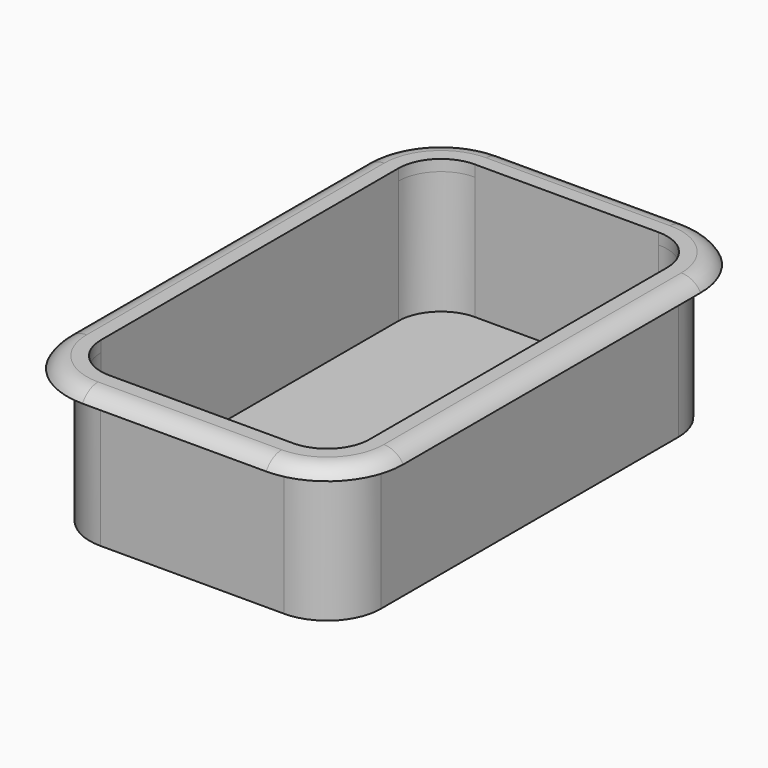
from build123d import *

# Parameters (mm, degrees)
F1_DEPTH     = 30
F2_T         = -2.5
F4_DEPTH     = 2.5
F5_T1_DEPTH  = 83
F5_T3_DEPTH  = 41
F5_T6_ANGLE  = 90
F5_T8_ANGLE  = 90
F5_T10_ANGLE = 90
F5_T12_ANGLE = 90


# Not quite as in the source:
# - a fillet or chamfer that OpenCascade refuses, or shapes differently, is made with other operations: its cross-section is extruded or revolved along the edge and cut away or added


with BuildPart() as f1:
    # F0 (on Top) → F1 (new body)
    with BuildSketch(Plane.XY):
        with BuildLine():
            ThreePointArc((32.5, 41.5), (28.9852813742, 49.9852813742), (20.5, 53.5))
            Line((20.5, 53.5), (-20.5, 53.5))
            ThreePointArc((-20.5, 53.5), (-28.9852813742, 49.9852813742), (-32.5, 41.5))
            Line((-32.5, 41.5), (-32.5, -41.5))
            ThreePointArc((-32.5, -41.5), (-28.9852813742, -49.9852813742), (-20.5, -53.5))
            Line((-20.5, -53.5), (20.5, -53.5))
            ThreePointArc((20.5, -53.5), (28.9852813742, -49.9852813742), (32.5, -41.5))
            Line((32.5, -41.5), (32.5, 41.5))
        make_face()
    extrude(amount=F1_DEPTH)

    # F2
    f2_openings = [f1.faces().sort_by_distance(p)[0] for p in [
        (0, 0, 30),
    ]]
    offset(amount=F2_T, openings=f2_openings)

    # F3 (on face) → F4 (join)
    with BuildSketch(Plane.XY.offset(30)):
        with BuildLine():
            Line((-20.5, -58.5), (20.5, -58.5))
            ThreePointArc((20.5, -58.5), (32.5208152802, -53.5208152802), (37.5, -41.5))
            Line((37.5, -41.5), (37.5, 41.5))
            ThreePointArc((37.5, 41.5), (32.5208152802, 53.5208152802), (20.5, 58.5))
            Line((20.5, 58.5), (-20.5, 58.5))
            ThreePointArc((-20.5, 58.5), (-32.5208152802, 53.5208152802), (-37.5, 41.5))
            Line((-37.5, 41.5), (-37.5, -41.5))
            ThreePointArc((-37.5, -41.5), (-32.5208152802, -53.5208152802), (-20.5, -58.5))
        make_face()
        with BuildLine():
            ThreePointArc((20.5, 53.5), (28.9852813742, 49.9852813742), (32.5, 41.5))
            Line((32.5, 41.5), (32.5, -41.5))
            ThreePointArc((32.5, -41.5), (28.9852813742, -49.9852813742), (20.5, -53.5))
            Line((20.5, -53.5), (-20.5, -53.5))
            ThreePointArc((-20.5, -53.5), (-28.9852813742, -49.9852813742), (-32.5, -41.5))
            Line((-32.5, -41.5), (-32.5, 41.5))
            ThreePointArc((-32.5, 41.5), (-28.9852813742, 49.9852813742), (-20.5, 53.5))
            Line((-20.5, 53.5), (20.5, 53.5))
        make_face(mode=Mode.SUBTRACT)
        with BuildLine():
            Line((32.5, -41.5), (32.5, 41.5))
            ThreePointArc((32.5, 41.5), (28.9852813742, 49.9852813742), (20.5, 53.5))
            Line((20.5, 53.5), (-20.5, 53.5))
            ThreePointArc((-20.5, 53.5), (-28.9852813742, 49.9852813742), (-32.5, 41.5))
            Line((-32.5, 41.5), (-32.5, -41.5))
            ThreePointArc((-32.5, -41.5), (-28.9852813742, -49.9852813742), (-20.5, -53.5))
            Line((-20.5, -53.5), (20.5, -53.5))
            ThreePointArc((20.5, -53.5), (28.9852813742, -49.9852813742), (32.5, -41.5))
        make_face()
        with BuildLine():
            Line((-20.5, 51), (20.5, 51))
            ThreePointArc((20.5, 51), (27.2175144213, 48.2175144213), (30, 41.5))
            Line((30, 41.5), (30, -41.5))
            ThreePointArc((30, -41.5), (27.2175144213, -48.2175144213), (20.5, -51))
            Line((20.5, -51), (-20.5, -51))
            ThreePointArc((-20.5, -51), (-27.2175144213, -48.2175144213), (-30, -41.5))
            Line((-30, -41.5), (-30, 41.5))
            ThreePointArc((-30, 41.5), (-27.2175144213, 48.2175144213), (-20.5, 51))
        make_face(mode=Mode.SUBTRACT)
    extrude(amount=F4_DEPTH)

    # F5: fillet of radius 5 on 1 edges, made by hand

    # F5_s2 → F5_t1 (cut)
    with BuildSketch(Plane.XZ.offset(-41.5)):
        with BuildLine():
            ThreePointArc((33.1698729811, 32.5), (35.6698729811, 31.8301270189), (37.5, 30))
            Line((37.5, 30), (37.5, 32.5))
            Line((37.5, 32.5), (33.1698729811, 32.5))
        make_face()
        with BuildLine():
            ThreePointArc((-33.1698729811, 32.5), (-35.6698729811, 31.8301270189), (-37.5, 30))
            Line((-37.5, 30), (-37.5, 32.5))
            Line((-37.5, 32.5), (-33.1698729811, 32.5))
        make_face()
    extrude(amount=F5_T1_DEPTH, mode=Mode.SUBTRACT)

    # F5_s4 → F5_t3 (cut)
    with BuildSketch(Plane.YZ.offset(-20.5)):
        with BuildLine():
            ThreePointArc((58.5, 30), (56.6698729811, 31.8301270189), (54.1698729811, 32.5))
            Line((54.1698729811, 32.5), (58.5, 32.5))
            Line((58.5, 32.5), (58.5, 30))
        make_face()
        with BuildLine():
            ThreePointArc((-54.1698729811, 32.5), (-56.6698729811, 31.8301270189), (-58.5, 30))
            Line((-58.5, 30), (-58.5, 32.5))
            Line((-58.5, 32.5), (-54.1698729811, 32.5))
        make_face()
    extrude(amount=F5_T3_DEPTH, mode=Mode.SUBTRACT)

    # F5_s5 → F5_t6 (revolve, cut)
    with BuildSketch(Plane.YZ.offset(20.5)):
        with BuildLine():
            ThreePointArc((-54.1698729811, 32.5), (-56.6698729811, 31.8301270189), (-58.5, 30))
            Line((-58.5, 30), (-58.5, 32.5))
            Line((-58.5, 32.5), (-54.1698729811, 32.5))
        make_face()
    revolve(axis=Axis((20.5, -41.5, 32.5), (0, 0, 1)), revolution_arc=F5_T6_ANGLE, mode=Mode.SUBTRACT)

    # F5_s7 → F5_t8 (revolve, cut)
    with BuildSketch(Plane.XZ.offset(-41.5)):
        with BuildLine():
            ThreePointArc((33.1698729811, 32.5), (35.6698729811, 31.8301270189), (37.5, 30))
            Line((37.5, 30), (37.5, 32.5))
            Line((37.5, 32.5), (33.1698729811, 32.5))
        make_face()
    revolve(axis=Axis((20.5, 41.5, 32.5), (0, 0, 1)), revolution_arc=F5_T8_ANGLE, mode=Mode.SUBTRACT)

    # F5_s9 → F5_t10 (revolve, cut)
    with BuildSketch(Plane.YZ.offset(-20.5)):
        with BuildLine():
            ThreePointArc((54.1698729811, 32.5), (56.6698729811, 31.8301270189), (58.5, 30))
            Line((58.5, 30), (58.5, 32.5))
            Line((58.5, 32.5), (54.1698729811, 32.5))
        make_face()
    revolve(axis=Axis((-20.5, 41.5, 32.5), (0, 0, 1)), revolution_arc=F5_T10_ANGLE, mode=Mode.SUBTRACT)

    # F5_s11 → F5_t12 (revolve, cut)
    with BuildSketch(Plane.XZ.offset(41.5)):
        with BuildLine():
            ThreePointArc((-33.1698729811, 32.5), (-35.6698729811, 31.8301270189), (-37.5, 30))
            Line((-37.5, 30), (-37.5, 32.5))
            Line((-37.5, 32.5), (-33.1698729811, 32.5))
        make_face()
    revolve(axis=Axis((-20.5, -41.5, 32.5), (0, 0, 1)), revolution_arc=F5_T12_ANGLE, mode=Mode.SUBTRACT)


solid = f1.part
